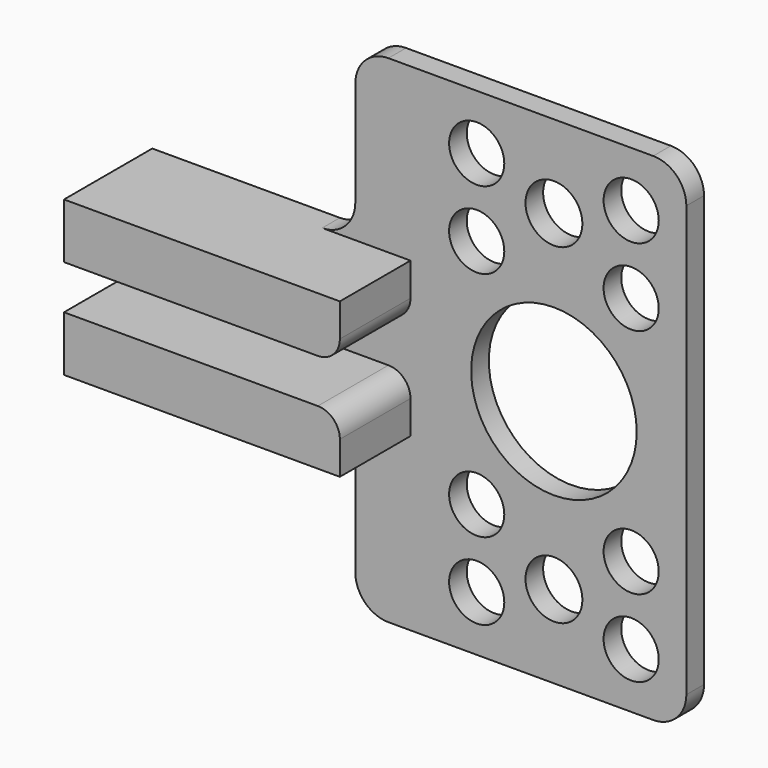
from build123d import *

# Parameters (mm, degrees)
F0_W      = 50
F0_H      = 10
F1_DEPTH  = 45
F2_R      = 2.5781
F3_DEPTH  = 25
F4_R      = 7.5
F5_DEPTH  = 10.001
F6_R      = 2.5
F7_DEPTH  = 25
F8_W      = 20
F8_H      = 15.5
F9_DEPTH  = 25
F8_R      = 2.5
F8_R_2    = 2.5781
F8_W_2    = 25
F8_H_2    = 4
F10_DEPTH = 8
F11_R     = 3
F12_R     = 2


# Not quite as in the source:
# - a feature of the source that left no trace in its solid (it failed there, or was rolled back) is left out


with BuildPart() as f1:
    # F0 (on Top) → F1 (new body)
    with BuildSketch(Plane.XY):
        Rectangle(F0_W, F0_H)
    extrude(amount=F1_DEPTH)

    # F2 (on face) → F3 (cut)
    with BuildSketch(Plane.XZ.offset(5)):
        with Locations((13, 37.5)):
            Circle(F2_R)
        with Locations((13, 7.5)):
            Circle(F2_R)
    extrude(amount=-F3_DEPTH, mode=Mode.SUBTRACT)

    # F4 (on face) → F5 (cut, through all)
    with BuildSketch(Plane.XZ.offset(5)):
        with Locations((13, 22.5)):
            Circle(F4_R)
    extrude(amount=-F5_DEPTH, mode=Mode.SUBTRACT)

    # F6 (on face) → F7 (cut)
    with BuildSketch(Plane.XZ.offset(5)):
        with Locations((6, 5)):
            Circle(F6_R)
        with Locations((6, 40)):
            Circle(F6_R)
        with Locations((20, 5)):
            Circle(F6_R)
        with Locations((20, 40)):
            Circle(F6_R)
        with Locations((6, 12)):
            Circle(F6_R)
        with Locations((6, 33)):
            Circle(F6_R)
        with Locations((20, 12)):
            Circle(F6_R)
        with Locations((20, 33)):
            Circle(F6_R)
    extrude(amount=-F7_DEPTH, mode=Mode.SUBTRACT)

    # F8 (on face) → F9 (cut)
    with BuildSketch(Plane.XZ.offset(5)):
        with Locations((-15, 7.75)):
            Rectangle(F8_W, F8_H)
        with Locations((-15, 37.25)):
            Rectangle(F8_W, F8_H)
    extrude(amount=-F9_DEPTH, mode=Mode.SUBTRACT)

    # F8 (on face) → F10 (cut)
    with BuildSketch(Plane.XZ.offset(5)):
        with BuildLine():
            Line((-5, 29.5), (0, 29.5))
            Line((0, 29.5), (10.3074175964, 29.5))
            ThreePointArc((10.3074175964, 29.5), (17.2459175671, 28.6824092402), (20.5, 22.5))
            ThreePointArc((20.5, 22.5), (17.2459175671, 16.3175907598), (10.3074175964, 15.5))
            Line((10.3074175964, 15.5), (0, 15.5))
            Line((0, 15.5), (-5, 15.5))
            Line((-5, 15.5), (-5, 0))
            Line((-5, 0), (25, 0))
            Line((25, 0), (25, 45))
            Line((25, 45), (-5, 45))
            Line((-5, 45), (-5, 29.5))
        make_face()
        with Locations((6, 5)):
            Circle(F8_R, mode=Mode.SUBTRACT)
        with Locations((20, 5)):
            Circle(F8_R, mode=Mode.SUBTRACT)
        with Locations((13, 7.5)):
            Circle(F8_R_2, mode=Mode.SUBTRACT)
        with Locations((6, 12)):
            Circle(F8_R, mode=Mode.SUBTRACT)
        with Locations((20, 12)):
            Circle(F8_R, mode=Mode.SUBTRACT)
        with Locations((6, 33)):
            Circle(F8_R, mode=Mode.SUBTRACT)
        with Locations((20, 33)):
            Circle(F8_R, mode=Mode.SUBTRACT)
        with Locations((6, 40)):
            Circle(F8_R, mode=Mode.SUBTRACT)
        with Locations((13, 37.5)):
            Circle(F8_R_2, mode=Mode.SUBTRACT)
        with Locations((20, 40)):
            Circle(F8_R, mode=Mode.SUBTRACT)
        with Locations((-12.5, 22.5)):
            Rectangle(F8_W_2, F8_H_2)
        with BuildLine():
            Line((10.3074175964, 24.5), (5.7715838526, 24.5))
            ThreePointArc((5.7715838526, 24.5), (5.5, 22.5), (5.7715838526, 20.5))
            Line((5.7715838526, 20.5), (10.3074175964, 20.5))
            Line((10.3074175964, 20.5), (10.3074175964, 24.5))
        make_face()
        with BuildLine():
            Line((5.7715838526, 20.5), (0, 20.5))
            Line((0, 20.5), (0, 15.5))
            Line((0, 15.5), (10.3074175964, 15.5))
            ThreePointArc((10.3074175964, 15.5), (7.4451324892, 17.4608089004), (5.7715838526, 20.5))
        make_face()
        with BuildLine():
            Line((5.7715838526, 24.5), (0, 24.5))
            Line((0, 24.5), (0, 20.5))
            Line((0, 20.5), (5.7715838526, 20.5))
            ThreePointArc((5.7715838526, 20.5), (5.5, 22.5), (5.7715838526, 24.5))
        make_face()
        with BuildLine():
            Line((0, 29.5), (0, 24.5))
            Line((0, 24.5), (5.7715838526, 24.5))
            ThreePointArc((5.7715838526, 24.5), (7.4451324892, 27.5391910996), (10.3074175964, 29.5))
            Line((10.3074175964, 29.5), (0, 29.5))
        make_face()
    extrude(amount=-F10_DEPTH, mode=Mode.SUBTRACT)

    # F11
    f11_edges = [f1.edges().sort_by_distance(p)[0] for p in [
        (25, 4, 0),
        (25, 4, 45),
        (-5, 4, 45),
        (-5, 4, 29.5),
        (-5, 4, 0),
        (-5, 4, 15.5),
    ]]
    fillet(f11_edges, radius=F11_R)

    # F12
    f12_edges = [f1.edges().sort_by_distance(p)[0] for p in [
        (0, -1, 20.5),
        (0, -1, 24.5),
    ]]
    fillet(f12_edges, radius=F12_R)


solid = f1.part
